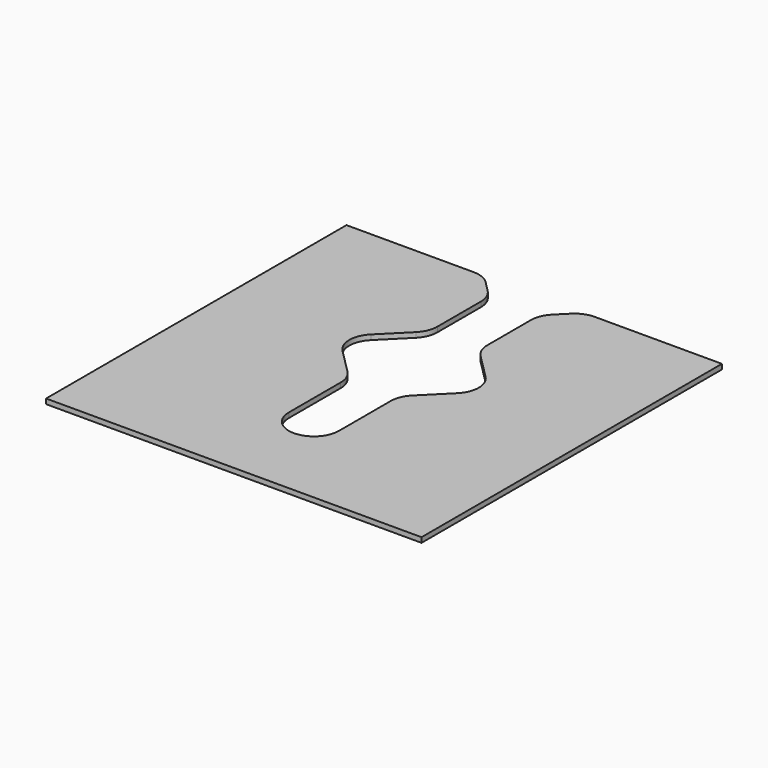
from build123d import *

# Parameters (mm, degrees)
F1_DEPTH = 4
F2_R     = 20
F3_R     = 19.99999


# Not quite as in the source:
# - a fillet or chamfer is up to 0.001 mm smaller than in the source, because OpenCascade refuses the exact size


with BuildPart() as f1:
    # F0 (on Top) → F1 (new body)
    with BuildSketch(Plane.XY):
        Polygon((0, 300), (0, 0), (150, 0), (150, 60), (130, 60), (130, 140), (90, 180), (130, 220), (130, 280), (110, 300), align=None)
        Polygon((150, 60), (150, 0), (300, 0), (300, 300), (190, 300), (170, 280), (170, 220), (210, 180), (170, 140), (170, 60), align=None)
    extrude(amount=F1_DEPTH)

    # F2
    f2_edges = [f1.edges().sort_by_distance(p)[0] for p in [
        (130, 60, 2),
        (130, 140, 2),
        (90, 180, 2),
        (130, 220, 2),
        (130, 280, 2),
        (110, 300, 2),
    ]]
    fillet(f2_edges, radius=F2_R)

    # F3 (radius 20 in the source; OpenCascade refuses exactly that, so slightly less here)
    f3_edges = [f1.edges().sort_by_distance(p)[0] for p in [
        (190, 300, 2),
        (170, 280, 2),
        (170, 220, 2),
        (210, 180, 2),
        (170, 140, 2),
        (170, 60, 2),
    ]]
    fillet(f3_edges, radius=F3_R)


solid = f1.part
